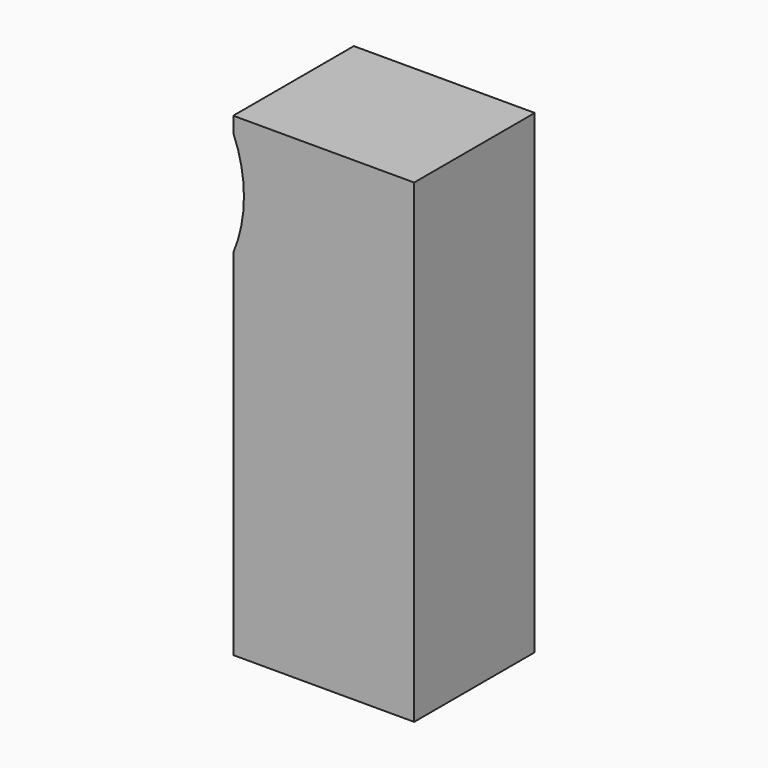
from build123d import *

# Parameters (mm, degrees)
F0_W     = 12
F0_H     = 31.5
F1_DEPTH = 10
F3_DEPTH = 10.001


# Not quite as in the source:
# - a feature names something its author has since deleted; it is built from what else it names


with BuildPart() as f1:
    # F0 (on Front) → F1 (new body)
    with BuildSketch(Plane.XZ):
        with Locations((6, 15.75)):
            Rectangle(F0_W, F0_H)
    extrude(amount=F1_DEPTH)

    # F2 (on face) → F3 (cut, through all)
    with BuildSketch(Plane.XZ.offset(10)):
        with BuildLine():
            Line((0, 30.5), (0, 23.5))
            ThreePointArc((0, 23.5), (0.7084380241, 27), (0, 30.5))
        make_face()
    extrude(amount=-F3_DEPTH, mode=Mode.SUBTRACT)


solid = f1.part
